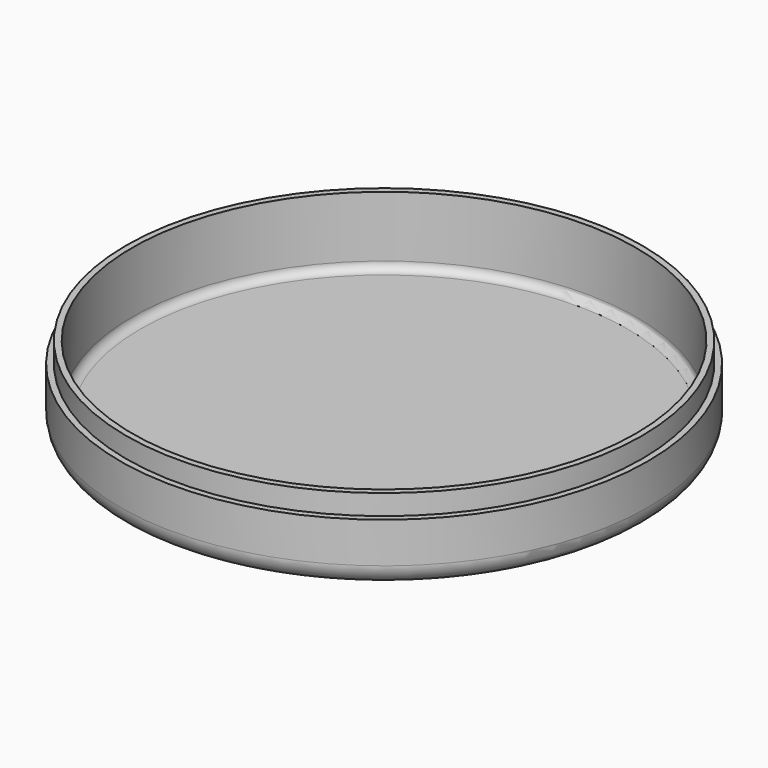
from build123d import *

# Parameters (mm, degrees)
F0_R     = 32.5
F1_DEPTH = 10
F2_R     = 2.5
F3_T     = -1.5
F4_R     = 32.5
F4_R_2   = 31.75
F5_DEPTH = 2.5


# Not quite as in the source:
# - a feature names something its author has since deleted; it is built from what else it names


with BuildPart() as f1:
    # F0 (on Top) → F1 (new body)
    with BuildSketch(Plane.XY):
        Circle(F0_R)
    extrude(amount=F1_DEPTH)

    # F2
    f2_edges = [f1.edges().sort_by_distance(p)[0] for p in [
        (-32.5, 0, 0),
    ]]
    fillet(f2_edges, radius=F2_R)

    # F3
    f3_openings = [f1.faces().sort_by_distance(p)[0] for p in [
        (0, 0, 10),
    ]]
    offset(amount=F3_T, openings=f3_openings)

    # F4 (on face) → F5 (cut)
    with BuildSketch(Plane.XY.offset(10)):
        Circle(F4_R)
        Circle(F4_R_2, mode=Mode.SUBTRACT)
    extrude(amount=-F5_DEPTH, mode=Mode.SUBTRACT)


solid = f1.part
